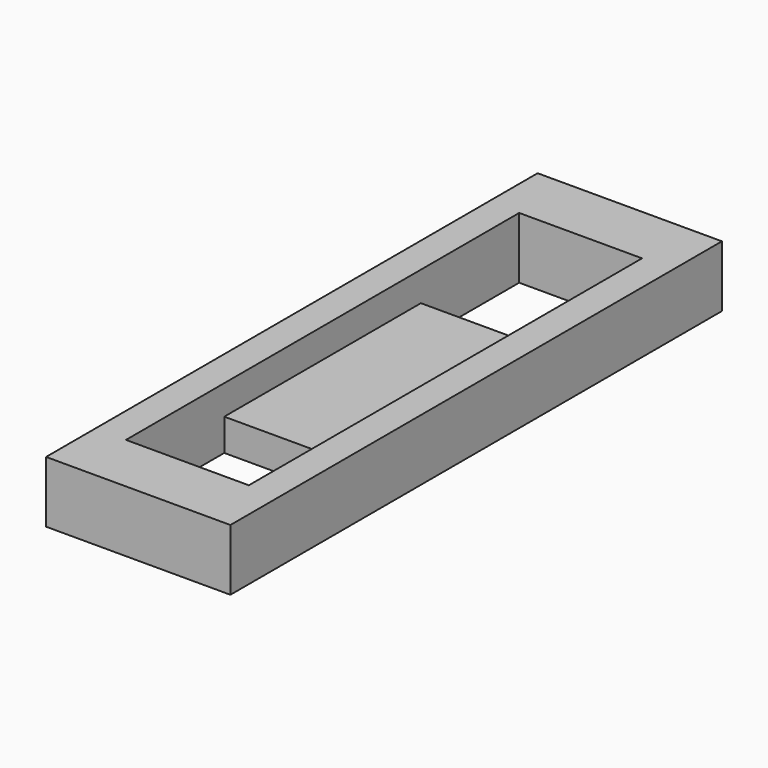
from build123d import *

# Parameters (mm, degrees)
F0_W     = 19.05
F0_H     = 63.5
F0_W_2   = 12.7
F0_H_2   = 50.8
F1_DEPTH = 6.35
F2_W     = 12.7
F2_H     = 25.4
F3_DEPTH = 3.302


# Not quite as in the source:
# - the program builds the solid bodies; features that only make, move or delete a surface that nothing else refers to are left out


with BuildPart() as f1:
    # F0 (on Top) → F1 (new body)
    with BuildSketch(Plane.XY):
        with Locations((-33.0491933286, -43.7945974991)):
            Rectangle(F0_W, F0_H)
        with Locations((-33.0491933286, -43.7945974991)):
            Rectangle(F0_W_2, F0_H_2, mode=Mode.SUBTRACT)
    extrude(amount=F1_DEPTH)

    # F2 (on Top) → F3 (join)
    with BuildSketch(Plane.XY):
        with Locations((-33.0491933286, -43.7945974991)):
            Rectangle(F2_W, F2_H)
    extrude(amount=F3_DEPTH)


solid = f1.part
